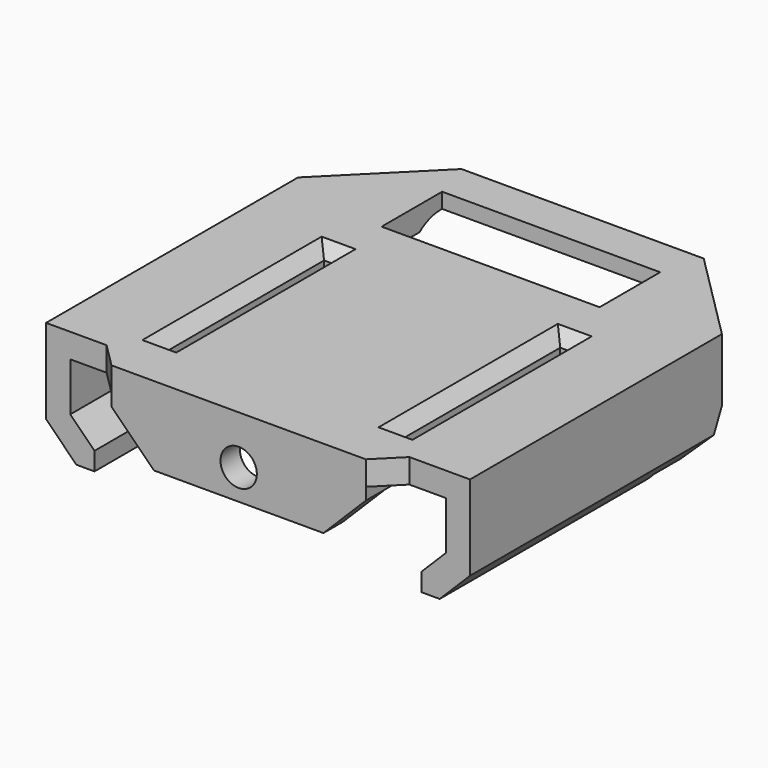
from build123d import *

# Parameters (mm, degrees)
F1_DEPTH  = 67
F3_DEPTH  = 70.001
F4_W      = 36
F4_H      = 12.5
F5_DEPTH  = 25
F6_W      = 3
F6_H      = 43
F7_DEPTH  = 2
F8_W      = 1.6
F8_H      = 33
F9_DEPTH  = 6.001
F10_W     = 42
F10_H     = 4
F11_DEPTH = 13
F13_SIZE  = 5
F14_SIZE  = 3.99999
F15_SIZE  = 15
F16_SIZE  = 7
F12_R     = 3
F17_DEPTH = 71.001
F18_W     = 30
F18_H     = 45
F19_DEPTH = 3
F20_SIZE  = 2.99999
F21_SIZE  = 2
F22_SIZE2 = 1.5
F22_SIZE  = 2.5
F24_START = -43
F23_W     = 62
F23_H     = 16.8932331726
F24_DEPTH = 57


# Not quite as in the source:
# - a fillet or chamfer is up to 0.001 mm smaller than in the source, because OpenCascade refuses the exact size


with BuildPart() as f1:
    # F0 (on Front) → F1 (new body)
    with BuildSketch(Plane.XZ):
        Polygon((35, 0), (-35, 0), (-35, -19), (-27, -19), (-27, -16), (-31, -12), (-31, -4), (31, -4), (31, -12), (27, -16), (27, -19), (35, -19), align=None)
    extrude(amount=F1_DEPTH)

    # F2 (on face) → F3 (cut, through all)
    with BuildSketch(Plane.YZ.offset(35)):
        with BuildLine():
            Line((-13.190586324, -6.5416721678), (-19, -19))
            Line((-19, -19), (4.1351475573, -19))
            Line((4.1351475573, -19), (4.1351475573, -2.5))
            Line((4.1351475573, -2.5), (-6.8464318148, -2.5))
            ThreePointArc((-6.8464318148, -2.5), (-10.6075290732, -3.5962598793), (-13.190586324, -6.5416721678))
        make_face()
    extrude(amount=-F3_DEPTH, mode=Mode.SUBTRACT)

    # F4 (on face) → F5 (cut)
    with BuildSketch(Plane.XY):
        with Locations((0, -12.75)):
            Rectangle(F4_W, F4_H)
    extrude(amount=-F5_DEPTH, mode=Mode.SUBTRACT)

    # F6 (on face) → F7 (join)
    with BuildSketch(Plane(origin=(0, 0, -4), x_dir=(1, 0, 0), z_dir=(0, 0, -1))):
        with Locations((-19.5, 45.5)):
            Rectangle(F6_W, F6_H)
        with Locations((19.5, 45.5)):
            Rectangle(F6_W, F6_H)
    extrude(amount=F7_DEPTH)

    # F8 (on face) → F9 (cut, through all)
    with BuildSketch(Plane(origin=(0, 0, -6), x_dir=(1, 0, 0), z_dir=(0, 0, -1))):
        with Locations((-19.5, 44.5)):
            Rectangle(F8_W, F8_H)
        with Locations((19.5, 44.5)):
            Rectangle(F8_W, F8_H)
    extrude(amount=-F9_DEPTH, mode=Mode.SUBTRACT)

    # F10 (on face) → F11 (join)
    with BuildSketch(Plane.XY):
        with Locations((0, -69)):
            Rectangle(F10_W, F10_H)
    extrude(amount=-F11_DEPTH)

    # F13
    f13_edges = [f1.edges().sort_by_distance(p)[0] for p in [
        (-35, -43, -19),
        (35, -43, -19),
    ]]
    chamfer(f13_edges, length=F13_SIZE)

    # F14 (size 4 in the source; OpenCascade refuses exactly that, so slightly less here)
    f14_edges = [f1.edges().sort_by_distance(p)[0] for p in [
        (-21, -67, -2),
        (21, -67, -2),
    ]]
    chamfer(f14_edges, length=F14_SIZE)

    # F15
    f15_edges = [f1.edges().sort_by_distance(p)[0] for p in [
        (35, 0, -1.25),
        (-35, 0, -1.25),
    ]]
    chamfer(f15_edges, length=F15_SIZE)

    # F16
    f16_edges = [f1.edges().sort_by_distance(p)[0] for p in [
        (-21, -69, -13),
        (21, -69, -13),
    ]]
    chamfer(f16_edges, length=F16_SIZE)

    # F12 (on face) → F17 (cut, through all)
    with BuildSketch(Plane.XZ.offset(71)):
        with Locations((0, -8)):
            Circle(F12_R)
    extrude(amount=-F17_DEPTH, mode=Mode.SUBTRACT)

    # F18 (on face) → F19 (cut)
    with BuildSketch(Plane(origin=(0, 0, -4), x_dir=(1, 0, 0), z_dir=(0, 0, -1))):
        with Locations((0, 44.5)):
            Rectangle(F18_W, F18_H)
    extrude(amount=-F19_DEPTH, mode=Mode.SUBTRACT)

    # F20 (size 3 in the source; OpenCascade refuses exactly that, so slightly less here)
    f20_edges = [f1.edges().sort_by_distance(p)[0] for p in [
        (0, -67, -1),
        (-15, -44.5, -1),
        (0, -22, -1),
        (15, -44.5, -1),
    ]]
    chamfer(f20_edges, length=F20_SIZE)

    # F21
    f21_edges = [f1.edges().sort_by_distance(p)[0] for p in [
        (20.3, -44.5, 0),
        (18.7, -44.5, 0),
        (19.5, -28, 0),
        (19.5, -61, 0),
        (-18.7, -44.5, 0),
        (-19.5, -28, 0),
        (-19.5, -61, 0),
        (-20.3, -44.5, 0),
    ]]
    chamfer(f21_edges, length=F21_SIZE)

    # F22
    f22_edges = [f1.edges().sort_by_distance(p)[0] for p in [
        (0, 0, -2.5),
    ]]
    f22_side = f1.faces().sort_by_distance((0, -3.465238, -2.5))[0]
    chamfer(f22_edges, length=F22_SIZE, length2=F22_SIZE2, reference=f22_side)

    # F23 (on face) → F24 (cut)
    with BuildSketch(Plane.XZ.offset(67).offset(F24_START)):
        with Locations((0, -17.7232683636)):
            Rectangle(F23_W, F23_H)
    extrude(amount=-F24_DEPTH, mode=Mode.SUBTRACT)


solid = f1.part
